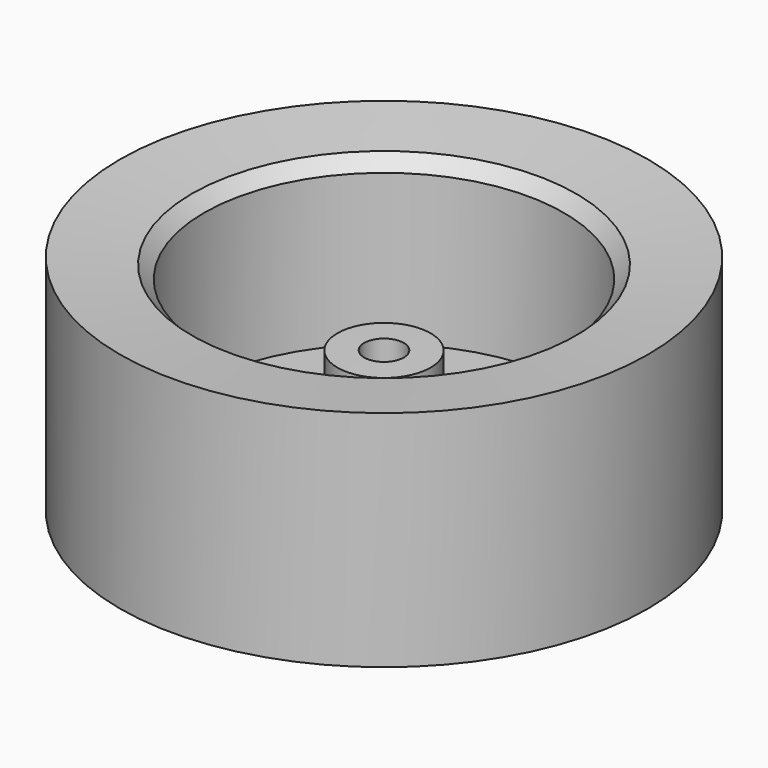
from build123d import *


# Not quite as in the source:
# - the program builds the solid bodies; features that only make, move or delete a surface that nothing else refers to are left out


with BuildPart() as f3:
    # F0 (on Front) → F3 (revolve)
    with BuildSketch(Plane.XZ):
        Polygon((-17.78, 15.0583637878), (-17.78, 13.335), (-17.78, 0), (0, 0), (0, 3.175), (-1.333490266, 3.1800951451), (-1.333490266, 9.5300951451), (-3.1368569799, 9.5191381732), (-3.1368569799, 3.1691381732), (-12.9158569799, 3.1691381732), (-12.9158569799, 13.3291381732), (-12.1086742729, 13.7421209365), (-12.9313254729, 14.6059049293), align=None)
    revolve(axis=Axis((0, 0, 1.5875), (0, 0, -1)))


solid = f3.part
